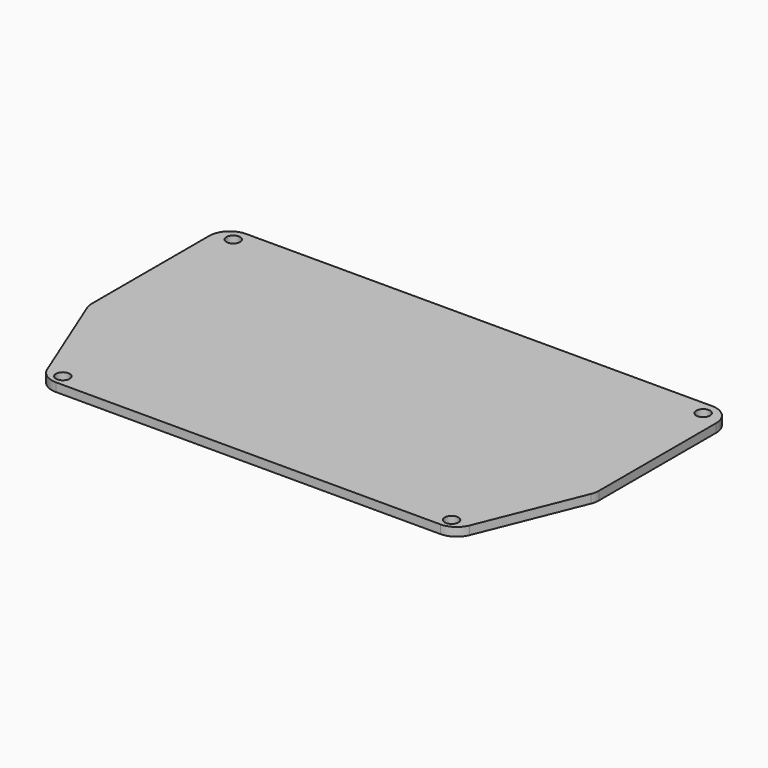
from build123d import *

# Parameters (mm, degrees)
F0_R     = 1
F1_DEPTH = 1.25
F2_R     = 3


with BuildPart() as f1:
    # F0 (on Top) → F1 (new body)
    with BuildSketch(Plane.XY):
        Polygon((0, 17.3524001093), (0, 42.3524001093), (-74, 42.3524001093), (-74, 17.3524001093), (-67.080681713, 0.2000030523), (-6.919318287, 0.2000030523), align=None)
        with Locations((-65.375, 1.8524001093)):
            Circle(F0_R, mode=Mode.SUBTRACT)
        with Locations((-8.625, 1.8524001093)):
            Circle(F0_R, mode=Mode.SUBTRACT)
        with Locations((-71.3, 40.3524001093)):
            Circle(F0_R, mode=Mode.SUBTRACT)
        with Locations((-2.7, 40.3524001093)):
            Circle(F0_R, mode=Mode.SUBTRACT)
    extrude(amount=F1_DEPTH)

    # F2
    f2_edges = [f1.edges().sort_by_distance(p)[0] for p in [
        (0, 42.3524, 0.625),
        (-74, 42.3524, 0.625),
        (-74, 17.3524, 0.625),
        (0, 17.3524, 0.625),
        (-6.919318, 0.200003, 0.625),
        (-67.080682, 0.200003, 0.625),
    ]]
    fillet(f2_edges, radius=F2_R)


solid = f1.part
